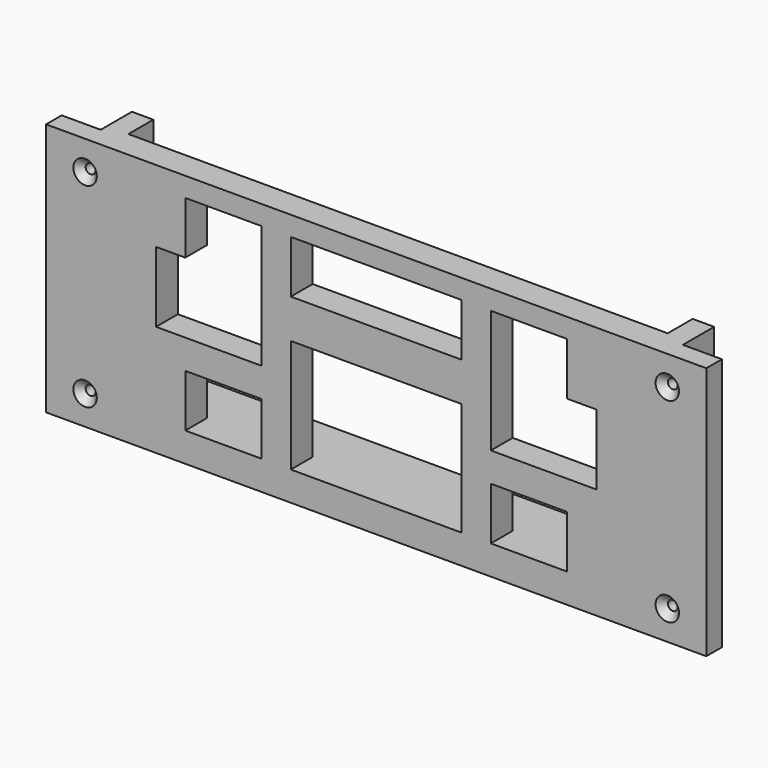
from build123d import *

# Parameters (mm, degrees)
F0_W      = 298.5
F0_H      = 130
F1_DEPTH  = 14
F2_W      = 20
F2_H      = 10
F3_DEPTH  = 130
F4_W      = 11
F4_H      = 16
F5_DEPTH  = 130
F6_W      = 39.1095238095
F6_H      = 26.9544340008
F6_W_2    = 43.7704761905
F6_H_2    = 58.0455659992
F7_DEPTH  = 25
F8_R      = 2.5
F9_DEPTH  = 25
F10_R     = 2.5
F11_DEPTH = 318.501
F12_SIZE  = 3.49999
F14_W     = 276.5
F14_H     = 15
F13_DEPTH = 25


# Not quite as in the source:
# - a fillet or chamfer is up to 0.001 mm smaller than in the source, because OpenCascade refuses the exact size
# - a feature names something its author has since deleted; it is built from what else it names


with BuildPart() as f1:
    # F0 (on Front) → F1 (new body)
    with BuildSketch(Plane.XZ):
        with Locations((149.25, 65)):
            Rectangle(F0_W, F0_H)
    extrude(amount=F1_DEPTH)

    # F2 (on face) → F3 (join, through all)
    with BuildSketch(Plane.XY.offset(130)):
        with Locations((308.5, -9)):
            Rectangle(F2_W, F2_H)
        with Locations((-10, -9)):
            Rectangle(F2_W, F2_H)
    extrude(amount=-F3_DEPTH)

    # F4 (on face) → F5 (join, through all)
    with BuildSketch(Plane.XY.offset(130)):
        with Locations((5.5, 8)):
            Rectangle(F4_W, F4_H)
        with Locations((293, 8)):
            Rectangle(F4_W, F4_H)
    extrude(amount=-F5_DEPTH)

    # F6 (on face) → F7 (cut)
    with BuildSketch(Plane.XZ.offset(14)):
        Polygon((51.37, 120), (51.37, 93.0455659992), (36.37, 93.0455659992), (36.3699999999, 56.9544340008), (90.4795238095, 56.9544340008), (90.4795238095, 120), align=None)
        with Locations((70.9247619048, 28.4772170004)):
            Rectangle(F6_W, F6_H)
        with Locations((127.3647619048, 44.0227829996)):
            Rectangle(F6_W_2, F6_H_2)
        with Locations((171.1352380952, 44.0227829996)):
            Rectangle(F6_W_2, F6_H_2)
        with Locations((127.3647619048, 106.5227829996)):
            Rectangle(F6_W_2, F6_H)
        with Locations((171.1352380952, 106.5227829996)):
            Rectangle(F6_W_2, F6_H)
        Polygon((247.1300000001, 120), (208.0204761905, 120), (208.0204761905, 56.9544340008), (262.13, 56.9544340008), (262.13, 93.0455659992), (247.13, 93.0455659992), align=None)
        with Locations((227.5752380952, 28.4772170004)):
            Rectangle(F6_W, F6_H)
    extrude(amount=-F7_DEPTH, mode=Mode.SUBTRACT)

    # F8 (on face) → F9 (cut)
    with BuildSketch(Plane(origin=(0, -4, 0), x_dir=(-1, 0, 0), z_dir=(0, 1, 0))):
        with Locations((-298.5, 115)):
            Circle(F8_R)
        with Locations((-298.5, 15)):
            Circle(F8_R)
        with Locations((0, 115)):
            Circle(F8_R)
        with Locations((0, 15)):
            Circle(F8_R)
    extrude(amount=-F9_DEPTH, mode=Mode.SUBTRACT)

    # F10 (on face) → F11 (cut, through all)
    with BuildSketch(Plane.YZ.offset(298.5)):
        with Locations((6, 115)):
            Circle(F10_R)
        with Locations((6, 15)):
            Circle(F10_R)
        with Locations((6, 65)):
            Circle(F10_R)
    extrude(amount=-F11_DEPTH, mode=Mode.SUBTRACT)

    # F12 (size 3.5 in the source; OpenCascade refuses exactly that, so slightly less here)
    f12_edges = [f1.edges().sort_by_distance(p)[0] for p in [
        (301, -14, 115),
        (301, -14, 15),
        (2.5, -14, 115),
        (2.5, -14, 15),
        (287.5, 3.5, 115),
        (287.5, 3.5, 65),
        (287.5, 3.5, 15),
        (11, 3.5, 115),
        (11, 3.5, 65),
        (11, 3.5, 15),
    ]]
    chamfer(f12_edges, length=F12_SIZE)

    # F14 (on face) → F13 (join)
    with BuildSketch(Plane(origin=(0, 0, 0), x_dir=(-1, 0, 0), z_dir=(0, 1, 0))):
        with Locations((-149.25, 7.5)):
            Rectangle(F14_W, F14_H)
    extrude(amount=F13_DEPTH)


solid = f1.part
